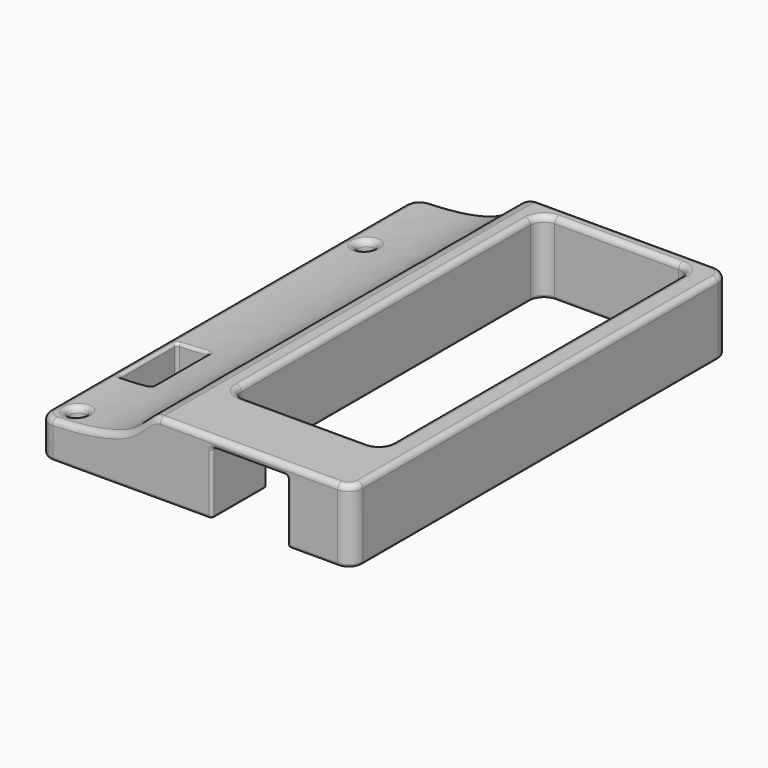
from build123d import *

# Parameters (mm, degrees)
F0_R     = 1.5
F1_DEPTH = 13
F3_DEPTH = 84.501
F4_W     = 13.5
F4_H     = 12.33
F4_H_2   = 4.67
F5_DEPTH = 11.3
F6_DEPTH = 13.0010001
F7_R     = 2.4
F8_W     = 6
F8_H     = 13
F9_DEPTH = 13.0010001
F10_R    = 0.5
F11_R    = 1
F12_R    = 1


with BuildPart() as f1:
    # F0 (on Top) → F1 (new body)
    with BuildSketch(Plane.XY):
        with BuildLine():
            ThreePointArc((28, 33.75), (27.267766953, 35.517766953), (25.5, 36.25))
            Line((25.5, 36.25), (-25.5, 36.25))
            ThreePointArc((-25.5, 36.25), (-27.267766953, 35.517766953), (-28, 33.75))
            Line((-28, 33.75), (-28, -33.75))
            ThreePointArc((-28, -33.75), (-27.267766953, -35.517766953), (-25.5, -36.25))
            Line((-25.5, -36.25), (25.5, -36.25))
            ThreePointArc((25.5, -36.25), (27.267766953, -35.517766953), (28, -33.75))
            Line((28, -33.75), (28, 33.75))
        make_face()
        with Locations((-24.25, -32.25)):
            Circle(F0_R, mode=Mode.SUBTRACT)
        with Locations((24.25, -32.25)):
            Circle(F0_R, mode=Mode.SUBTRACT)
        with Locations((-24.25, 32.25)):
            Circle(F0_R, mode=Mode.SUBTRACT)
        with Locations((24.25, 32.25)):
            Circle(F0_R, mode=Mode.SUBTRACT)
        with BuildLine():
            Line((-25.5, 36.25), (25.5, 36.25))
            ThreePointArc((25.5, 36.25), (27.267766953, 35.517766953), (28, 33.75))
            Line((28, 33.75), (28, 45.75))
            ThreePointArc((28, 45.75), (27.267766953, 47.517766953), (25.5, 48.25))
            Line((25.5, 48.25), (-25.5, 48.25))
            ThreePointArc((-25.5, 48.25), (-27.267766953, 47.517766953), (-28, 45.75))
            Line((-28, 45.75), (-28, 33.75))
            ThreePointArc((-28, 33.75), (-27.267766953, 35.517766953), (-25.5, 36.25))
        make_face()
        with Locations((24.25, 32.25)):
            Circle(F0_R)
        with Locations((24.25, -32.25)):
            Circle(F0_R)
    extrude(amount=F1_DEPTH)

    # F2 (on face) → F3 (cut, through all)
    with BuildSketch(Plane.XZ.offset(36.25)):
        with BuildLine():
            add(Edge.make_bspline(
                [(-6.2572634779, 13), (-8.4680945771, 13), (-10.8106237918, 6.7341257295), (-25.5, 6.5), (-28, 6.5)],
                knots=[0, 0, 0, 0, 0.4063937774, 1, 1, 1, 1], degree=3))
            Line((-6.2572634779, 13), (-28, 13))
            Line((-28, 13), (-28, 6.5))
        make_face()
    extrude(amount=-F3_DEPTH, mode=Mode.SUBTRACT)

    # F4 (on face) → F5 (cut)
    with BuildSketch(Plane(origin=(0, 0, 0), x_dir=(1, 0, 0), z_dir=(0, 0, -1))):
        with Locations((9.75, 30.085)):
            Rectangle(F4_W, F4_H)
        with Locations((9.75, 21.585)):
            Rectangle(F4_W, F4_H_2)
    extrude(amount=-F5_DEPTH, mode=Mode.SUBTRACT)

    # F4 (on face) → F6 (cut, through all)
    with BuildSketch(Plane(origin=(0, 0, 0), x_dir=(1, 0, 0), z_dir=(0, 0, -1))):
        Polygon((16.5, 19.25), (3, 19.25), (3, 23.92), (-3.5, 23.92), (-3.5, -45.58), (23.5, -45.58), (23.5, 23.92), (16.5, 23.92), align=None)
        with Locations((9.75, 21.585)):
            Rectangle(F4_W, F4_H_2)
    extrude(amount=-F6_DEPTH, mode=Mode.SUBTRACT)

    # F7
    f7_edges = [f1.edges().sort_by_distance(p)[0] for p in [
        (-3.5, 45.58, 6.5),
        (23.5, 45.58, 6.5),
        (23.5, -23.92, 6.5),
        (-3.5, -23.92, 6.5),
    ]]
    fillet(f7_edges, radius=F7_R)

    # F8 (on face) → F9 (cut, through all)
    with BuildSketch(Plane(origin=(0, 0, 0), x_dir=(1, 0, 0), z_dir=(0, 0, -1))):
        with Locations((-23.5, 13.75)):
            Rectangle(F8_W, F8_H)
    extrude(amount=-F9_DEPTH, mode=Mode.SUBTRACT)

    # F10
    f10_edges = [f1.edges().sort_by_distance(p)[0] for p in [
        (3, -23.92, 5.65),
        (16.5, -23.92, 5.65),
        (3, -36.25, 5.65),
        (16.5, -36.25, 5.65),
        (18.8, -23.92, 0),
        (22.797056, -23.217056, 0),
        (16.5, -30.085, 0),
        (23.5, 10.83, 0),
        (21, -36.25, 0),
        (22.797056, 44.877056, 0),
        (27.267767, -35.517767, 0),
        (10, 45.58, 0),
        (28, 6, 0),
        (-2.797056, 44.877056, 0),
        (27.267767, 47.517767, 0),
        (-3.5, 10.83, 0),
        (0, 48.25, 0),
        (-2.797056, -23.217056, 0),
        (-27.267767, 47.517767, 0),
        (0.95, -23.92, 0),
        (-28, 6, 0),
        (3, -30.085, 0),
        (-27.267767, -35.517767, 0),
        (-11.25, -36.25, 0),
        (-25.75, -32.25, 0),
        (-20.5, -13.75, 0),
        (-23.5, -7.25, 0),
        (-26.5, -13.75, 0),
        (-23.5, -20.25, 0),
        (-25.75, 32.25, 0),
        (-20.5, -7.25, 3.44831),
        (-26.5, -7.25, 3.257947),
        (-26.5, -20.25, 3.257947),
        (-20.5, -20.25, 3.44831),
        (-26.5, -13.75, 6.515894),
        (16.5, -30.085, 11.3),
        (3, -30.085, 11.3),
        (9.75, -23.92, 11.3),
        (9.75, -36.25, 11.3),
        (-20.5, -13.75, 6.896619),
        (-23.496064, -7.25, 6.639101),
        (-23.496064, -20.25, 6.639101),
    ]]
    fillet(f10_edges, radius=F10_R)

    # F11
    f11_edges = [f1.edges().sort_by_distance(p)[0] for p in [
        (9.621368, -36.25, 13),
    ]]
    fillet(f11_edges, radius=F11_R)

    # F12
    f12_edges = [f1.edges().sort_by_distance(p)[0] for p in [
        (-2.797056, -23.217056, 13),
        (-22.75, -32.25, 3.594748),
        (-25.75, -32.25, 0.5),
        (-25.75, -32.25, 6.53523),
        (-22.75, 32.25, 3.594748),
        (-25.75, 32.25, 0.5),
        (-25.75, 32.25, 6.53523),
        (-3.5, 10.83, 13),
        (-2.797056, 44.877056, 13),
        (10, 45.58, 13),
        (10, -23.92, 13),
        (22.797056, 44.877056, 13),
        (22.797056, -23.217056, 13),
        (23.5, 10.83, 13),
    ]]
    fillet(f12_edges, radius=F12_R)


solid = f1.part
